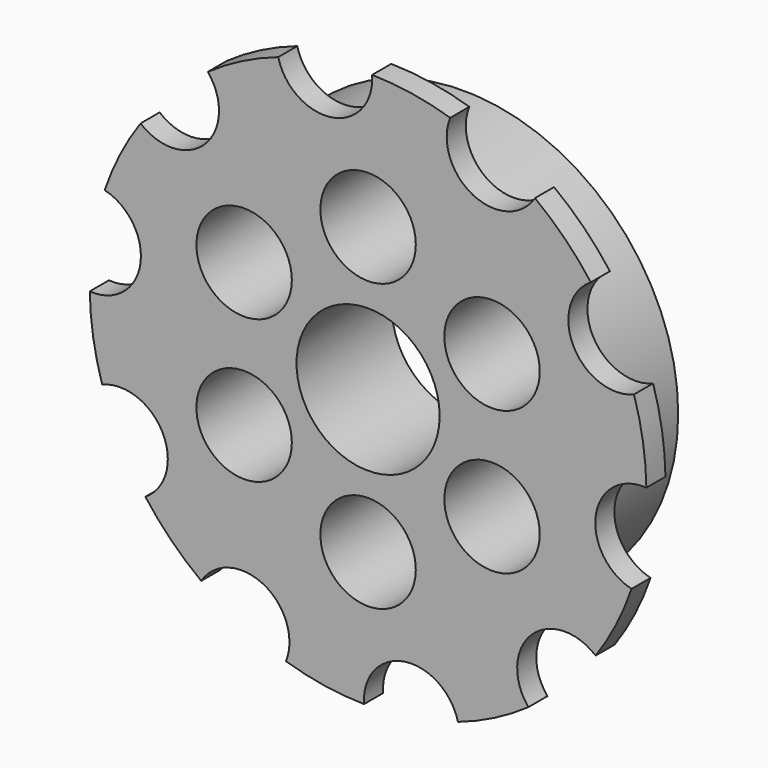
from build123d import *

# Parameters (mm, degrees)
F0_R     = 27
F1_DEPTH = 15
F2_R     = 35
F2_R_2   = 27
F3_DEPTH = 3
F4_R     = 9
F5_DEPTH = 15.001
F6_R     = 6
F7_DEPTH = 15.001


with BuildPart() as f1:
    # F0 (on Front) → F1 (new body)
    with BuildSketch(Plane.XZ):
        Circle(F0_R)
    extrude(amount=-F1_DEPTH)

    # F2 (on face) → F3 (join)
    with BuildSketch(Plane.XZ):
        Circle(F2_R)
        Circle(F2_R_2, mode=Mode.SUBTRACT)
    extrude(amount=-F3_DEPTH)

    # F4 (on face) → F5 (cut, through all)
    with BuildSketch(Plane.XZ):
        Circle(F4_R)
    extrude(amount=-F5_DEPTH, mode=Mode.SUBTRACT)

    # F6 (on face) → F7 (cut, through all)
    with BuildSketch(Plane.XZ):
        with Locations((0, 18)):
            Circle(F6_R)
        with Locations((-15.5884572681, 9)):
            Circle(F6_R)
        with Locations((-15.5884572681, -9)):
            Circle(F6_R)
        with Locations((0, -18)):
            Circle(F6_R)
        with BuildLine():
            ThreePointArc((-28.6121091704, 20.1580556806), (-22.2169623686, 19.3090576187), (-18.7487373415, 24.7487373415))
            ThreePointArc((-18.7487373415, 24.7487373415), (-19.1120676703, 26.8049365092), (-20.1580556806, 28.6121091704))
            ThreePointArc((-20.1580556806, 28.6121091704), (-24.7487373415, 24.7487373415), (-28.6121091704, 20.1580556806))
        make_face()
        with BuildLine():
            ThreePointArc((0.5095661882, 34.9962904077), (-5.4752062764, 34.5690919208), (-11.2990747198, 33.1259854265))
            ThreePointArc((-11.2990747198, 33.1259854265), (-4.7482986689, 28.6132875813), (0.5247937236, 34.5690919208))
            ThreePointArc((0.5247937236, 34.5690919208), (0.5209856313, 34.782826818), (0.5095661882, 34.9962904077))
        make_face()
        with BuildLine():
            ThreePointArc((-34.9962904077, -0.5095661882), (-34.5690919208, 5.4752062764), (-33.1259854265, 11.2990747198))
            ThreePointArc((-33.1259854265, 11.2990747198), (-40.4952219644, 6.4138130666), (-34.9962904077, -0.5095661882))
        make_face()
        with BuildLine():
            ThreePointArc((-28.5690919208, 5.4752062764), (-29.8437009864, 9.1725946137), (-33.1259854265, 11.2990747198))
            ThreePointArc((-33.1259854265, 11.2990747198), (-34.5690919208, 5.4752062764), (-34.9962904077, -0.5095661882))
            ThreePointArc((-34.9962904077, -0.5095661882), (-30.4802773568, 1.084124922), (-28.5690919208, 5.4752062764))
        make_face()
        with BuildLine():
            ThreePointArc((20.9825510926, 28.0130781894), (15.8896674909, 31.1852283466), (10.3298222323, 33.4409146503))
            ThreePointArc((10.3298222323, 33.4409146503), (13.1657244924, 25.8391892015), (20.9825510926, 28.0130781894))
        make_face()
        with BuildLine():
            ThreePointArc((-25.1852283466, -15.8896674909), (-27.8336703374, -10.9130161156), (-33.4409146503, -10.3298222323))
            ThreePointArc((-33.4409146503, -10.3298222323), (-31.1852283466, -15.8896674909), (-28.0130781894, -20.9825510926))
            ThreePointArc((-28.0130781894, -20.9825510926), (-25.9396158493, -18.8023208394), (-25.1852283466, -15.8896674909))
        make_face()
        with BuildLine():
            ThreePointArc((33.4409146503, 10.3298222323), (31.1852283466, 15.8896674909), (28.0130781894, 20.9825510926))
            ThreePointArc((28.0130781894, 20.9825510926), (25.8391892015, 13.1657244924), (33.4409146503, 10.3298222323))
        make_face()
        with BuildLine():
            ThreePointArc((37.1852283466, 15.8896674909), (34.0978816951, 21.1352799882), (28.0130781894, 20.9825510926))
            ThreePointArc((28.0130781894, 20.9825510926), (31.1852283466, 15.8896674909), (33.4409146503, 10.3298222323))
            ThreePointArc((33.4409146503, 10.3298222323), (36.1618797219, 12.5381094817), (37.1852283466, 15.8896674909))
        make_face()
        with BuildLine():
            ThreePointArc((-9.8896674909, -31.1852283466), (-14.2400162566, -25.4164632443), (-20.9825510926, -28.0130781894))
            ThreePointArc((-20.9825510926, -28.0130781894), (-15.8896674909, -31.1852283466), (-10.3298222323, -33.4409146503))
            ThreePointArc((-10.3298222323, -33.4409146503), (-10.00073416, -32.3343428858), (-9.8896674909, -31.1852283466))
        make_face()
        with BuildLine():
            ThreePointArc((35, 0), (34.9990725896, 0.2547898454), (34.9962904077, 0.5095661882))
            ThreePointArc((34.9962904077, 0.5095661882), (28.6429618773, -4.5365994862), (33.1259854265, -11.2990747198))
            ThreePointArc((33.1259854265, -11.2990747198), (34.5283180153, -5.726714157), (35, 0))
        make_face()
        with BuildLine():
            ThreePointArc((40.5690919208, -5.4752062764), (38.9601732752, -1.3863917123), (34.9962904077, 0.5095661882))
            ThreePointArc((34.9962904077, 0.5095661882), (34.9990725896, 0.2547898454), (35, 0))
            ThreePointArc((35, 0), (34.5283180153, -5.726714157), (33.1259854265, -11.2990747198))
            ThreePointArc((33.1259854265, -11.2990747198), (38.2664802582, -10.2005972108), (40.5690919208, -5.4752062764))
        make_face()
        with BuildLine():
            ThreePointArc((11.2990747198, -33.1259854265), (4.5365994862, -28.6429618773), (-0.5095661882, -34.9962904077))
            ThreePointArc((-0.5095661882, -34.9962904077), (5.4752062764, -34.5690919208), (11.2990747198, -33.1259854265))
        make_face()
        with BuildLine():
            ThreePointArc((20.1580556806, -28.6121091704), (24.7487373415, -24.7487373415), (28.6121091704, -20.1580556806))
            ThreePointArc((28.6121091704, -20.1580556806), (20.5060966544, -20.5060966544), (20.1580556806, -28.6121091704))
        make_face()
        with Locations((15.5884572681, -9)):
            Circle(F6_R)
        with Locations((15.5884572681, 9)):
            Circle(F6_R)
    extrude(amount=-F7_DEPTH, mode=Mode.SUBTRACT)


solid = f1.part
